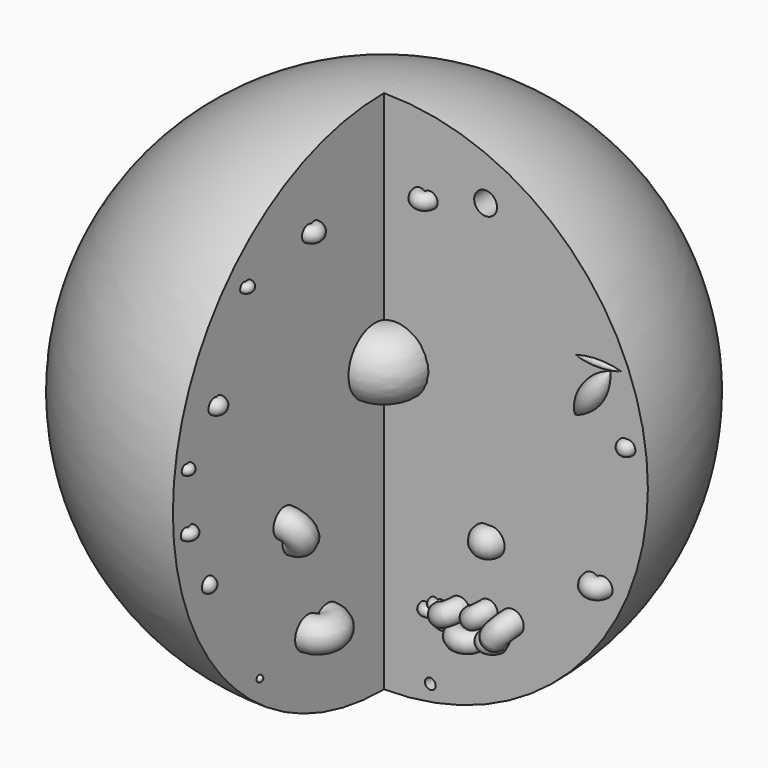
from build123d import *

# Parameters (mm, degrees)
F1_ANGLE  = 270
F24_R     = 0.5173814018
F25_DEPTH = 5
F26_R     = 1.1047616538
F27_DEPTH = 5


# Not quite as in the source:
# - the program builds the solid bodies; features that only make, move or delete a surface that nothing else refers to are left out


with BuildPart() as f1:
    # F0 (on Front) → F1 (revolve)
    with BuildSketch(Plane.XZ):
        with BuildLine():
            Line((0, 50.8), (0, 0))
            ThreePointArc((0, 0), (25.538163478, 25.4), (0, 50.8))
        make_face()
    revolve(axis=Axis((0, 0, 25.4), (0, 0, 1)), revolution_arc=F1_ANGLE)

    # F6 (on face) → F7 (revolve)
    with BuildSketch(Plane.XZ):
        with BuildLine():
            Line((10.1037621498, 17.2790959477), (10.1037621498, 14.6444309503))
            ThreePointArc((10.1037621498, 14.6444309503), (11.6720624424, 15.961763449), (10.1037621498, 17.2790959477))
        make_face()
    revolve(axis=Axis((10.1037621498, 0, 15.961763449), (0, 0, 1)))

    # F8 (on face) → F9 (revolve)
    with BuildSketch(Plane.YZ):
        with BuildLine():
            Line((-21.3061086833, 18.3257050812), (-21.3061086833, 16.8832316995))
            ThreePointArc((-21.3061086833, 16.8832316995), (-20.5848719925, 17.6044683903), (-21.3061086833, 18.3257050812))
        make_face()
    revolve(axis=Axis((0, -21.3061086833, 17.6044683903), (0, 0, 1)))

    # F10 (on face) → F11 (revolve)
    with BuildSketch(Plane.YZ):
        with BuildLine():
            Line((-16.6967175901, 41.531920433), (-16.6967175901, 40.7127737999))
            ThreePointArc((-16.6967175901, 40.7127737999), (-15.9933074588, 41.1223471165), (-16.6967175901, 41.531920433))
        make_face()
    revolve(axis=Axis((0, -16.6967175901, 41.1223471165), (0, 0, 1)))

    # F12 (on face) → F13 (revolve)
    with BuildSketch(Plane.YZ):
        with BuildLine():
            Line((-15.0985233486, 7.3720696382), (-15.0985233486, 6.7783878185))
            ThreePointArc((-15.0985233486, 6.7783878185), (-14.7831806465, 7.0752287284), (-15.0985233486, 7.3720696382))
        make_face()
    revolve(axis=Axis((0, -15.0985233486, 7.0752287284), (0, 0, 1)))

    # F24 (on face) → F25 (cut)
    with BuildSketch(Plane.XZ):
        with Locations((4.4794678688, 1.9284766167)):
            Circle(F24_R)
    extrude(amount=-F25_DEPTH, mode=Mode.SUBTRACT)

    # F26 (on face) → F27 (cut)
    with BuildSketch(Plane.XZ):
        with Locations((9.8344683647, 44.6154624224)):
            Circle(F26_R)
    extrude(amount=-F27_DEPTH, mode=Mode.SUBTRACT)

    # F28 (on face) → F29 (revolve)
    with BuildSketch(Plane.XZ):
        with BuildLine():
            Line((4.3995565746, 8.5433159037), (4.3995565746, 8.0433159037))
            ThreePointArc((4.3995565746, 8.0433159037), (5.3325692765, 8.2933159037), (4.3995565746, 8.5433159037))
        make_face()
    revolve(axis=Axis((4.3995565746, 0, 8.2933159037), (0, 0, 1)))

    # F30 (on face) → F31 (revolve)
    with BuildSketch(Plane.XZ):
        with BuildLine():
            Line((5.1990970969, 9.3276202679), (5.1990970969, 8.6431186646))
            ThreePointArc((5.1990970969, 8.6431186646), (6.0197488074, 8.9853694662), (5.1990970969, 9.3276202679))
        make_face()
    revolve(axis=Axis((5.1990970969, 0, 8.9853694662), (0, 0, 1)))

    # F32 (on face) → F33 (revolve)
    with BuildSketch(Plane.XZ):
        with BuildLine():
            ThreePointArc((5.721292961, 7.8672324459), (6.7622374855, 7.3057549246), (5.9679847498, 8.1821025165))
            Line((5.9679847498, 8.1821025165), (5.721292961, 7.8672324459))
        make_face()
    revolve(axis=Axis((5.8446388554, 0, 8.0246674812), (-0.6167294719, 0, -0.7871751765)))

    # F34 (on face) → F35 (revolve)
    with BuildSketch(Plane.XZ):
        with BuildLine():
            Line((6.3005497155, 9.308727928), (6.7972990253, 8.4408338543))
            ThreePointArc((6.7972990253, 8.4408338543), (8.1684367597, 9.8017277226), (6.3005497155, 9.308727928))
        make_face()
    revolve(axis=Axis((6.5489243704, 0, 8.8747808912), (-0.4967493098, 0, 0.8678940737)))

    # F36 (on face) → F37 (revolve)
    with BuildSketch(Plane.XZ):
        with BuildLine():
            ThreePointArc((8.029088378, 6.5558589995), (9.8459018418, 7.1539692581), (8.029088378, 7.7520795166))
            Line((8.029088378, 7.7520795166), (8.029088378, 6.5558589995))
        make_face()
    revolve(axis=Axis((8.029088378, 0, 7.1539692581), (0, 0, -1)))

    # F38 (on face) → F39 (revolve)
    with BuildSketch(Plane.XZ):
        with BuildLine():
            Line((9.1234480117, 9.9425915007), (9.7133511788, 9.1351175052))
            ThreePointArc((9.7133511788, 9.1351175052), (10.8290444149, 10.5694063864), (9.1234480117, 9.9425915007))
        make_face()
    revolve(axis=Axis((9.4183995953, 0, 9.5388545029), (-0.5899031672, 0, 0.8074739955)))

    # F40 (on face) → F41 (revolve)
    with BuildSketch(Plane.XZ):
        with BuildLine():
            Line((10.4977339506, 8.0424901098), (10.4977339506, 7.006207481))
            ThreePointArc((10.4977339506, 7.006207481), (11.8678686144, 7.5243487954), (10.4977339506, 8.0424901098))
        make_face()
    revolve(axis=Axis((10.4977339506, 0, 7.5243487954), (0, 0, 1)))

    # F42 (on face) → F43 (revolve)
    with BuildSketch(Plane.XZ):
        with BuildLine():
            Line((11.3880634308, 9.2558329925), (12.0636820793, 8.6858104914))
            ThreePointArc((12.0636820793, 8.6858104914), (13.1201359886, 10.6233709656), (11.3880634308, 9.2558329925))
        make_face()
    revolve(axis=Axis((11.7258727551, 0, 8.970821742), (-0.7643086194, 0, 0.6448506295)))

    # F46 (on face) → F47 (revolve)
    with BuildSketch(Plane.YZ):
        with BuildLine():
            Line((-20.3042030334, 33.1616699696), (-20.3042030334, 31.7816697061))
            ThreePointArc((-20.3042030334, 31.7816697061), (-19.3745247831, 32.4716698378), (-20.3042030334, 33.1616699696))
        make_face()
    revolve(axis=Axis((0, -20.3042030334, 32.4716698378), (0, 0, 1)))

    # F48 (on face) → F49 (revolve)
    with BuildSketch(Plane.YZ):
        with BuildLine():
            ThreePointArc((-23.7102285028, 23.4250985086), (-24.5820095381, 23.013452068), (-23.7102285028, 22.6018056273))
            Line((-23.7102285028, 22.6018056273), (-23.7102285028, 23.4250985086))
        make_face()
    revolve(axis=Axis((0, -23.7102285028, 23.013452068), (0, 0, 1)))

    # F50 (on face) → F51 (revolve)
    with BuildSketch(Plane.XZ):
        with BuildLine():
            Line((20.640514791, 16.3614749908), (20.640514791, 14.8583753034))
            ThreePointArc((20.640514791, 14.8583753034), (22.1127376672, 15.6099251471), (20.640514791, 16.3614749908))
        make_face()
    revolve(axis=Axis((20.640514791, 0, 15.6099251471), (0, 0, 1)))

    # F52 (on face) → F53 (revolve)
    with BuildSketch(Plane.XZ):
        with BuildLine():
            Line((23.4837681055, 28.959363699), (23.4837681055, 27.5857187808))
            ThreePointArc((23.4837681055, 27.5857187808), (24.3276339526, 28.2725412399), (23.4837681055, 28.959363699))
        make_face()
    revolve(axis=Axis((23.4837681055, 0, 28.2725412399), (0, 0, 1)))

    # F54 (on face) → F55 (revolve)
    with BuildSketch(Plane.XZ):
        with BuildLine():
            Line((21.9182521105, 34.2343002558), (18.5068845749, 29.4268280268))
            ThreePointArc((18.5068845749, 29.4268280268), (21.0650598212, 31.2256388051), (21.9182521105, 34.2343002558))
        make_face()
    revolve(axis=Axis((20.2125683427, 0, 31.8305641413), (0.5787033498, 0, 0.8155381248)))

    # F56 (on face) → F57 (revolve)
    with BuildSketch(Plane.XZ):
        with BuildLine():
            ThreePointArc((23.0017080903, 34.5460660756), (20.7794010639, 34.8573416432), (18.5570940375, 34.5460660756))
            Line((18.5570940375, 34.5460660756), (23.0017080903, 34.5460660756))
        make_face()
    revolve(axis=Axis((20.7794010639, 0, 34.5460660756), (1, 0, 0)))


with BuildPart() as f3:
    # F2 (on face) → F3 (revolve)
    with BuildSketch(Plane.YZ):
        with BuildLine():
            ThreePointArc((0, 31.4789116383), (-4.2957633905, 28.4394558191), (0, 25.4))
            Line((0, 25.4), (0, 31.4789116383))
        make_face()
    revolve(axis=Axis((0, 0, 28.4394558191), (0, 0, 1)))


with BuildPart() as f15:
    # F14 (on face) → F15 (revolve)
    with BuildSketch(Plane.YZ):
        with BuildLine():
            Line((-23.8164365292, 28.9061143994), (-23.8164365292, 28.0481427908))
            ThreePointArc((-23.8164365292, 28.0481427908), (-23.1624587624, 28.4771285951), (-23.8164365292, 28.9061143994))
        make_face()
    revolve(axis=Axis((0, -23.8164365292, 28.4771285951), (0, 0, 1)))


with BuildPart() as f17:
    # F16 (on face) → F17 (revolve)
    with BuildSketch(Plane.YZ):
        with BuildLine():
            ThreePointArc((-8.0109834671, 9.5950383693), (-10.7476444216, 8.5745677352), (-8.0109834671, 7.5540971011))
            Line((-8.0109834671, 7.5540971011), (-8.0109834671, 9.5950383693))
        make_face()
    revolve(axis=Axis((0, -8.0109834671, 8.5745677352), (0, 0, 1)))


with BuildPart() as f19:
    # F18 (on face) → F19 (revolve)
    with BuildSketch(Plane.YZ):
        with BuildLine():
            ThreePointArc((-10.683324188, 18.666613847), (-12.7165142958, 20.2692462615), (-12.1970772743, 17.7330132574))
            Line((-12.1970772743, 17.7330132574), (-10.683324188, 18.666613847))
        make_face()
    revolve(axis=Axis((0, -11.4402007312, 18.1998135522), (0, 0.8511408442, 0.5249373899)))


with BuildPart() as f21:
    # F20 (on face) → F21 (revolve)
    with BuildSketch(Plane.YZ):
        with BuildLine():
            ThreePointArc((-8.7961498648, 43.2516001165), (-9.9205043099, 42.5809789449), (-8.7961498648, 41.9103577733))
            Line((-8.7961498648, 41.9103577733), (-8.7961498648, 43.2516001165))
        make_face()
    revolve(axis=Axis((0, -8.7961498648, 42.5809789449), (0, 0, 1)))


with BuildPart() as f23:
    # F22 (on face) → F23 (revolve)
    with BuildSketch(Plane.XZ):
        with BuildLine():
            Line((3.9467960596, 43.7163822353), (3.9467960596, 42.5657443702))
            ThreePointArc((3.9467960596, 42.5657443702), (5.1955028438, 43.1410633028), (3.9467960596, 43.7163822353))
        make_face()
    revolve(axis=Axis((3.9467960596, 0, 43.1410633028), (0, 0, 1)))


solid = Compound([f1.part, f3.part, f15.part, f17.part, f19.part, f21.part, f23.part])
